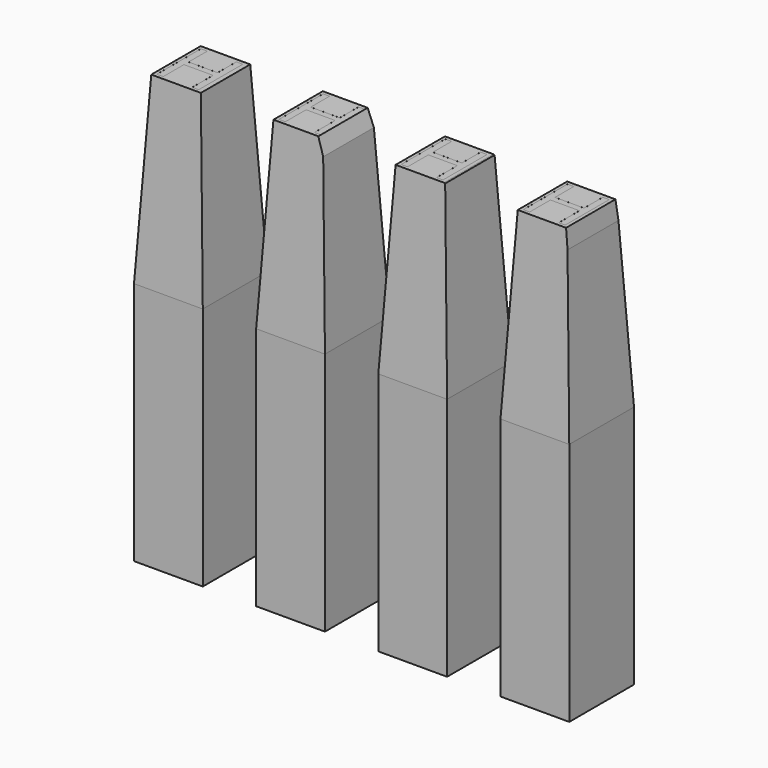
from build123d import *

# Parameters (mm, degrees)
F0_W         = 7.150608
F0_H         = 8.41248
F1_DEPTH     = 25.4
F1_FACE_W    = 7.150608
F1_FACE_H    = 8.41248
F2_DEPTH     = 19.05
F2_TAPER     = 3
F3_TEXT_SIZE = 8.0264873557
F4_DEPTH     = 0.00254
F10_DEPTH    = 8.41348
F13_DEPTH    = 8.41348
F16_DEPTH    = 8.41348


# Not quite as in the source:
# - Text() gives the source's letters only with a copy of the font that has no kerning and outlines rounded to 1/6400 em; it was checked with that copy


with BuildPart() as f1:
    # F0 (on Top) → F1 (new body)
    with BuildSketch(Plane.XY):
        with Locations((3.575304, 4.20624)):
            Rectangle(F0_W, F0_H)
    extrude(amount=-F1_DEPTH)

    # F1_face (on face) → F2 (join)
    with BuildSketch(Plane(origin=(3.575304, 4.20624, 0), x_dir=(1, 0, 0), z_dir=(0, 0, 1))):
        Rectangle(F1_FACE_W, F1_FACE_H)
    extrude(amount=F2_DEPTH, taper=F2_TAPER)

    # F3 (on face) → F4 (cut)
    with BuildSketch(Plane.XY.offset(19.05)):
        with Locations((0.5230585812, 1.32543582)):
            Text('H', F3_TEXT_SIZE, font='Open Sans', text_align=(TextAlign.LEFT, TextAlign.BOTTOM))
    extrude(amount=-F4_DEPTH, mode=Mode.SUBTRACT)


with BuildPart() as f6_1:
    # F6: copy of F1
    add(f1.part.moved(Location((12.7, 0, 0))))


with BuildPart() as f8_1:
    # F8: copy of F1
    add(f1.part.moved(Location((12.7, 0, 0))))

    # F9 (on Front) → F10 (cut, through all)
    with BuildSketch(Plane.XZ):
        Polygon((19.0266477681, 19.05), (18.3612646275, 19.05), (19.0266477681, 17.145), align=None)
    extrude(amount=-F10_DEPTH, mode=Mode.SUBTRACT)


with BuildPart() as f11_1:
    # F11: copy of F1
    add(f1.part.moved(Location((25.4, 0, 0))))

    # F12 (on Front) → F13 (cut, through all)
    with BuildSketch(Plane.XZ):
        Polygon((32.394554466, 19.2665141076), (30.8481473476, 19.1866997629), (32.394554466, 18.8175588846), align=None)
    extrude(amount=-F13_DEPTH, mode=Mode.SUBTRACT)


with BuildPart() as f14_1:
    # F14: copy of F11_1
    add(f11_1.part.moved(Location((12.7, 0, 0))))

    # F15 (on Front) → F16 (cut, through all)
    with BuildSketch(Plane.XZ):
        Polygon((44.3520766242, 19.0812298009), (44.120810791, 19.05), (44.3520766242, 17.145), align=None)
    extrude(amount=-F16_DEPTH, mode=Mode.SUBTRACT)


solid = Compound([f1.part, f8_1.part, f11_1.part, f14_1.part])
